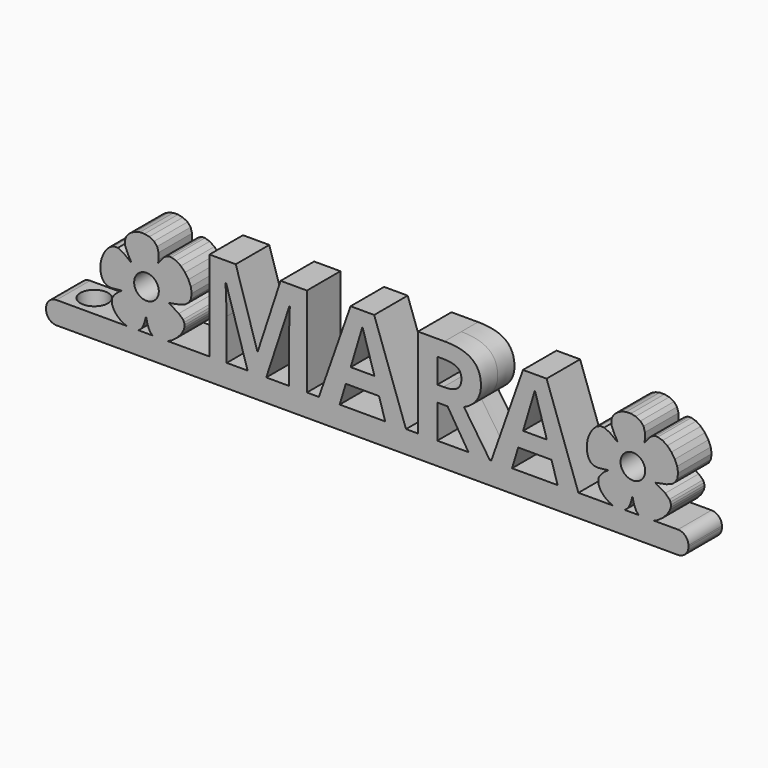
from build123d import *

# Parameters (mm, degrees)
F0_R         = 1.7660260944
F0_TEXT_SIZE = 18.2894468259
F1_DEPTH     = 3
F2_W         = 84.5
F2_H         = 6
F3_DEPTH     = 0.2
F4_DEPTH     = 3
F5_W         = 6
F5_H         = 3.2
F6_DEPTH     = 7.5
F7_R         = 1.5
F8_R         = 2
F9_DEPTH     = 4
F10_R        = 1.5


# Not quite as in the source:
# - Text() gives the source's letters only with a copy of the font that has no kerning and outlines rounded to 1/6400 em; it was checked with that copy


with BuildPart() as f1:
    # F0 (on Front) → F1 (new body, symmetric)
    with BuildSketch(Plane.XZ):
        Polygon((-9.8962181259, -0.0299609487), (-9.3093152472, 0.0995427735), (-8.5310452338, 0.4643787281), (-7.7886221935, 1.0156229815), (-7.1753136859, 1.6703047867), (-6.7844076966, 2.345448762), (-6.6844409889, 2.697736103), (-6.6652413988, 3.0240118702), (-6.7312263226, 3.3305926174), (-6.8868132072, 3.6238062576), (-7.4844896445, 4.1953846804), (-8.4936258745, 4.789299945), (-8.9274018823, 5.0567831788), (-8.4181052429, 5.1580766137), (-7.3131137554, 5.3695361907), (-6.5480905692, 5.6521941874), (-6.0523445823, 6.043851435), (-5.7552051187, 6.5823041299), (-5.6420905942, 7.3346827833), (-5.7751165223, 8.1369112107), (-6.1089634595, 8.9328581362), (-6.5983028952, 9.6663968681), (-7.1978267956, 10.281407439), (-7.8622157172, 10.7217585729), (-8.546147975, 10.9313258196), (-8.8812811082, 10.9320270148), (-9.2043064176, 10.8539824368), (-9.6469000392, 10.5612860557), (-10.1400767255, 9.9810366231), (-10.4508130024, 9.5801644376), (-10.4068223535, 10.0271686751), (-10.3916193646, 10.9311557532), (-10.598433195, 11.6324207168), (-11.0363252865, 12.1480644274), (-11.7143548393, 12.4951945719), (-12.3982545289, 12.6383143795), (-13.0712303381, 12.6247535348), (-13.7032208938, 12.4733707309), (-14.2641853, 12.2030313855), (-14.7240621838, 11.8325941916), (-15.0528129411, 11.3809291004), (-15.2203761991, 10.8668948051), (-15.1967042361, 10.3093544817), (-14.8286469794, 9.4077545862), (-14.3529716358, 8.5454741101), (-14.2906102139, 8.4004774316), (-14.4811582303, 8.5293860258), (-15.3946726039, 9.2300894295), (-16.21802192, 9.6332437342), (-16.8030362894, 9.634121823), (-17.3568401554, 9.3699870508), (-17.8525159958, 8.8932532172), (-18.2631576982, 8.2563454299), (-18.5618432066, 7.5116797807), (-18.7216618753, 6.7116836696), (-18.7156984739, 5.9087754295), (-18.5170445979, 5.1553756349), (-18.2008868091, 4.6439944488), (-17.7512302174, 4.3560670179), (-17.1086136552, 4.2712956407), (-16.2135760559, 4.3694053341), (-15.7044514474, 4.4302814773), (-15.6696932647, 4.4000047008), (-15.7790195709, 4.3290260096), (-16.1651405309, 4.0708069691), (-16.5523139664, 3.7127982689), (-16.8671052824, 3.3322639471), (-17.0360798838, 3.0064680418), (-17.0831036318, 2.6043628391), (-17.0239245605, 2.1921008316), (-16.867618816, 1.7819255621), (-16.6232807801, 1.3860941234), (-16.3000002503, 1.0168545414), (-15.9068693162, 0.6864593752), (-15.4529754831, 0.4071521172), (-14.9474063577, 0.1911989779), (-14.4397479673, 0.0570083052), (-13.9840845603, 0.0188926715), (-13.5797273957, 0.0772799851), (-13.2259605822, 0.2326232662), (-12.9220907946, 0.485341356), (-12.6674066752, 0.8358849825), (-12.4612081239, 1.2846821047), (-12.3027905578, 1.8321743328), (-12.1879723822, 2.2557758958), (-12.1309056827, 2.0998483864), (-12.0112204133, 1.5291342486), (-11.8237778137, 0.9902805659), (-11.5954117235, 0.5466869075), (-11.3529559319, 0.2617414835), (-10.9521058183, 0.053843468), (-10.4551700276, -0.0442881949), align=None)
        with Locations((-12.1185852993, 6.0541479067)):
            Circle(F0_R, mode=Mode.SUBTRACT)
        Polygon((59.526901838, 9.9810366231), (59.2161655612, 9.5801644376), (59.26015621, 10.0271686751), (59.2753591989, 10.9311557532), (59.0685453685, 11.6324207168), (58.6306532771, 12.1480644274), (57.9526237243, 12.4951945719), (57.2687240346, 12.6383143795), (56.5957482255, 12.6247535348), (55.9637576698, 12.4733707309), (55.4027932636, 12.2030313855), (54.9429163798, 11.8325941916), (54.6141656224, 11.3809291004), (54.4466023644, 10.8668948051), (54.4702743274, 10.3093544817), (54.8383315841, 9.4077545862), (55.3140069277, 8.5454741101), (55.3763683496, 8.4004774316), (55.1858203332, 8.5293860258), (54.2723059597, 9.2300894295), (53.4489566436, 9.6332437342), (52.8639422742, 9.634121823), (52.3101384081, 9.3699870508), (51.8144625677, 8.8932532172), (51.4038208654, 8.2563454299), (51.1051353569, 7.5116797807), (50.9453166883, 6.7116836696), (50.9512800897, 5.9087754295), (51.1499339657, 5.1553756349), (51.4660917545, 4.6439944488), (51.9157483462, 4.3560670179), (52.5583649084, 4.2712956407), (53.4534025077, 4.3694053341), (53.9625271162, 4.4302814773), (53.9972852989, 4.4000047008), (53.8879589927, 4.3290260096), (53.5018380327, 4.0708069691), (53.1146645972, 3.7127982689), (52.7998732812, 3.3322639471), (52.6308986797, 3.0064680418), (52.5838749317, 2.6043628391), (52.6430540031, 2.1921008316), (52.7993597475, 1.7819255621), (53.0436977834, 1.3860941234), (53.3669783132, 1.0168545414), (53.7601092474, 0.6864593752), (54.2140030805, 0.4071521172), (54.7195722058, 0.1911989779), (55.2272305962, 0.0570083052), (55.6828940033, 0.0188926715), (56.0872511678, 0.0772799851), (56.4410179814, 0.2326232662), (56.7448877689, 0.485341356), (56.9995718883, 0.8358849825), (57.2057704397, 1.2846821047), (57.3641880058, 1.8321743328), (57.4790061813, 2.2557758958), (57.5360728808, 2.0998483864), (57.6557581502, 1.5291342486), (57.8432007498, 0.9902805659), (58.07156684, 0.5466869075), (58.3140226317, 0.2617414835), (58.7148727453, 0.053843468), (59.211808536, -0.0442881949), (59.7707604376, -0.0299609487), (60.3576633164, 0.0995427735), (61.1359333298, 0.4643787281), (61.87835637, 1.0156229815), (62.4916648777, 1.6703047867), (62.8825708669, 2.345448762), (62.9825375747, 2.697736103), (63.0017371647, 3.0240118702), (62.9357522409, 3.3305926174), (62.7801653564, 3.6238062576), (62.1824889191, 4.1953846804), (61.173352689, 4.789299945), (60.7395766813, 5.0567831788), (61.2488733207, 5.1580766137), (62.3538648082, 5.3695361907), (63.1188879943, 5.6521941874), (63.6146339812, 6.043851435), (63.9117734448, 6.5823041299), (64.0248879693, 7.3346827833), (63.8918620412, 8.1369112107), (63.558015104, 8.9328581362), (63.0686756684, 9.6663968681), (62.4691517679, 10.281407439), (61.8047628464, 10.7217585729), (61.1208305885, 10.9313258196), (60.7856974553, 10.9320270148), (60.462672146, 10.8539824368), (60.0200785243, 10.5612860557), align=None)
        with Locations((57.5483932642, 6.0541479067)):
            Circle(F0_R, mode=Mode.SUBTRACT)
        with Locations((-4.742804654, 0)):
            Text('MARA', F0_TEXT_SIZE, font='Open Sans', font_style=FontStyle.BOLD, text_align=(TextAlign.LEFT, TextAlign.BOTTOM))
    extrude(amount=F1_DEPTH, both=True)



with BuildPart() as f3:
    # F2 (on Top) → F3 (new body)
    with BuildSketch(Plane.XY):
        with Locations((23.25, 0)):
            Rectangle(F2_W, F2_H)
    extrude(amount=F3_DEPTH)


with BuildPart() as f4:
    # F4 (new): a face of the model
    f4_faces = [f3.part.faces().sort_by_distance(p)[0] for p in [
        (23.25, 0, 0),
    ]]
    extrude(f4_faces, amount=F4_DEPTH)


with BuildPart() as f1_1:
    add(f1.part)

    add(f3.part)  # F6 merges F3

    add(f4.part)  # F6 merges F4
    # F5 (on face) → F6 (join)
    with BuildSketch(Plane(origin=(-19, 0, 0), x_dir=(0, -1, 0), z_dir=(-1, 0, 0))):
        with Locations((0, -1.4)):
            Rectangle(F5_W, F5_H)
    extrude(amount=F6_DEPTH)

    # F7
    f7_edges = [f1_1.edges().sort_by_distance(p)[0] for p in [
        (-26.5, 0, -3),
        (-26.5, 0, 0.2),
        (65.5, 0, -3),
    ]]
    fillet(f7_edges, radius=F7_R)

    # F8 (on face) → F9 (cut)
    with BuildSketch(Plane.XY.offset(0.2)):
        with Locations((-22, 0)):
            Circle(F8_R)
    extrude(amount=-F9_DEPTH, mode=Mode.SUBTRACT)

    # F10
    f10_edges = [f1_1.edges().sort_by_distance(p)[0] for p in [
        (65.5, 0, 0.2),
    ]]
    fillet(f10_edges, radius=F10_R)


solid = f1_1.part
